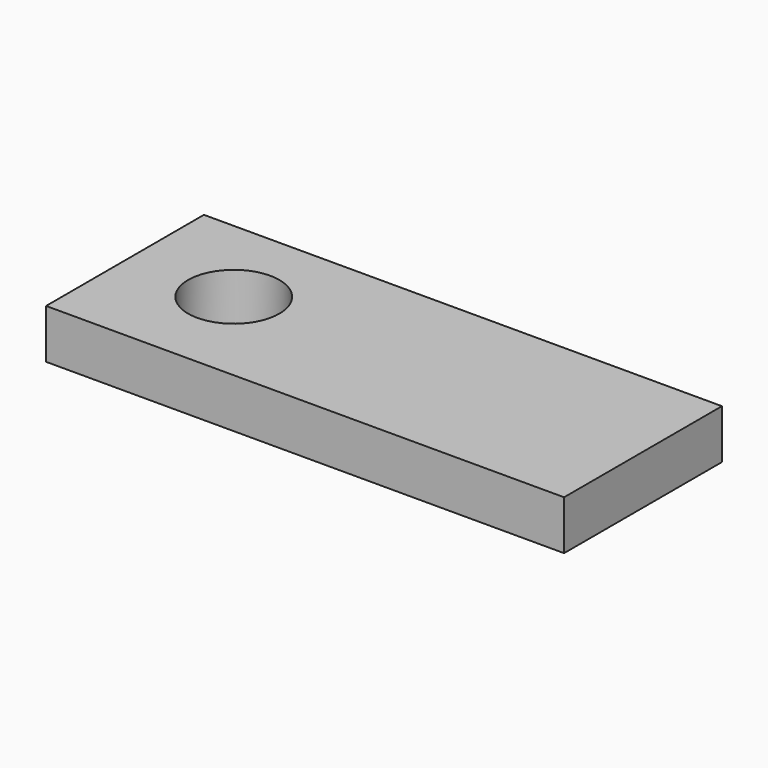
from build123d import *

# Parameters (mm, degrees)
F0_W     = 133.6440593004
F0_H     = 50.9024597704
F0_R     = 11.7707327429
F1_DEPTH = 12.7


# Not quite as in the source:
# - a feature names something its author has since deleted; it is built from what else it names


with BuildPart() as f1:
    # F0 (on Top) → F1 (new body)
    with BuildSketch(Plane.XY):
        with Locations((66.8220296502, -25.4512298852)):
            Rectangle(F0_W, F0_H)
        with Locations((27.039218694, -24.171281606)):
            Circle(F0_R, mode=Mode.SUBTRACT)
    extrude(amount=F1_DEPTH)


solid = f1.part
